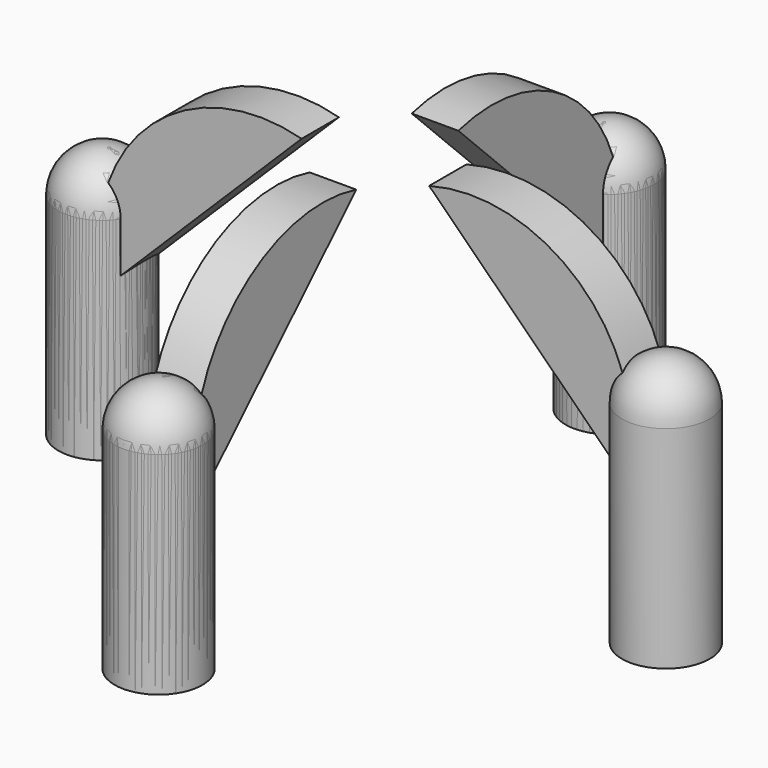
from build123d import *

# Parameters (mm, degrees)
F0_W          = 3.3492567
F0_H          = 16.1260536
F3_COUNT      = 4
F6_DEPTH      = 1.778
F6_DEPTH_BACK = 1.778
F7_COUNT      = 4


# Not quite as in the source:
# - a feature of the source that left no trace in its solid (it failed there, or was rolled back) is left out
# - a feature names something its author has since deleted; it is built from what else it names
# - the program builds the solid bodies; features that only make, move or delete a surface that nothing else refers to are left out


with BuildPart() as f2:
    # F0 (on Front) → F2 (revolve)
    with BuildSketch(Plane.XZ):
        with Locations((3.261367252, -32.3810689361)):
            Rectangle(F0_W, F0_H)
        with BuildLine():
            Line((-1.762517798, -24.3180421361), (1.586738902, -24.3180421361))
            Line((1.586738902, -24.3180421361), (1.586738902, -20.9687854361))
            ThreePointArc((1.586738902, -20.9687854361), (-0.7815432225, -21.9497600116), (-1.762517798, -24.3180421361))
        make_face()
    revolve(axis=Axis((1.586738902, 0, -19.72339442), (0, 0, 1)))


with BuildPart() as f3_1:
    # F3: instance of F2
    add(f2.part.rotate(Axis((-19.9247309591, 0, -2.3128986359), (0, 0, -1)), 1 * 360 / F3_COUNT))


with BuildPart() as f3_2:
    # F3: instance of F2
    add(f2.part.rotate(Axis((-19.9247309591, 0, -2.3128986359), (0, 0, -1)), 2 * 360 / F3_COUNT))


with BuildPart() as f3_3:
    # F3: instance of F2
    add(f2.part.rotate(Axis((-19.9247309591, 0, -2.3128986359), (0, 0, -1)), 3 * 360 / F3_COUNT))


with BuildPart() as f2_1:
    add(f2.part)

    # F5 (on Front) → F6 (join, two sides)
    with BuildSketch(Plane.XZ) as f6_sk:
        with BuildLine():
            Line((-15.0563139468, -14.4341522828), (0, -29.3660350144))
            ThreePointArc((0, -29.3660350144), (-3.2239997966, -17.5600688241), (-15.0563139468, -14.4341522828))
        make_face()
    extrude(amount=F6_DEPTH)
    extrude(f6_sk.sketch, amount=-F6_DEPTH_BACK)


with BuildPart() as f7_1:
    # F7: instance of F2
    add(f2_1.part.rotate(Axis((-19.9247309591, 0, -2.3128986359), (0, 0, -1)), 1 * 360 / F7_COUNT))


with BuildPart() as f7_2:
    # F7: instance of F2
    add(f2_1.part.rotate(Axis((-19.9247309591, 0, -2.3128986359), (0, 0, -1)), 2 * 360 / F7_COUNT))


with BuildPart() as f7_3:
    # F7: instance of F2
    add(f2_1.part.rotate(Axis((-19.9247309591, 0, -2.3128986359), (0, 0, -1)), 3 * 360 / F7_COUNT))


solid = Compound([f3_1.part, f3_2.part, f3_3.part, f2_1.part, f7_1.part, f7_2.part, f7_3.part])
